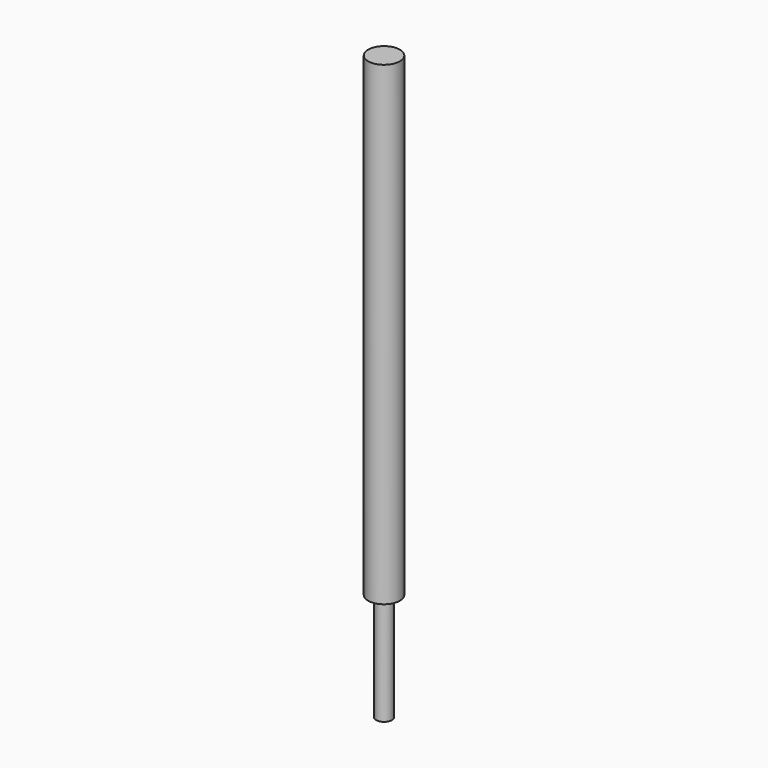
from build123d import *

# Parameters (mm, degrees)
F0_R     = 2.54
F1_DEPTH = 38.1
F2_R     = 1.27
F3_DEPTH = 17.272


# Not quite as in the source:
# - the program builds the solid bodies; features that only make, move or delete a surface that nothing else refers to are left out


with BuildPart() as f1:
    # F0 (on Top) → F1 (new body, symmetric)
    with BuildSketch(Plane.XY):
        Circle(F0_R)
    extrude(amount=F1_DEPTH, both=True)

    # F2 (on face) → F3 (join, symmetric)
    with BuildSketch(Plane(origin=(0, 0, -38.1), x_dir=(1, 0, 0), z_dir=(0, 0, -1))):
        Circle(F2_R)
    extrude(amount=F3_DEPTH, both=True)


solid = f1.part
